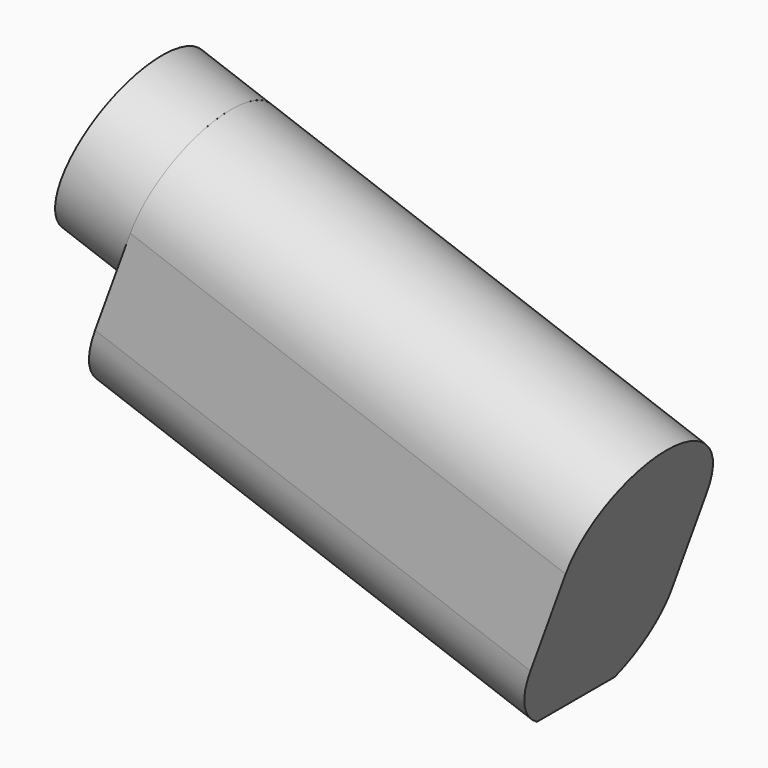
from build123d import *

# Parameters (mm, degrees)
F4_START = 63
F4_DEPTH = 10
F5_DEPTH = 63


# Not quite as in the source:
# - the program builds the solid bodies; features that only make, move or delete a surface that nothing else refers to are left out


with BuildPart() as f4:
    # F3 (on line) → F4 (new body)
    with BuildSketch(Plane(origin=(0, 0, 0), x_dir=(0, -1, 0), z_dir=(-0.9396926208, 0, 0.3420201433)).offset(F4_START)):
        with BuildLine():
            ThreePointArc((-12, 0), (0, -12), (12, 0))
            ThreePointArc((12, 0), (0, 12), (-12, 0))
        make_face()
    extrude(amount=F4_DEPTH)


with BuildPart() as f5:
    # F3 (on line) → F5 (new body)
    with BuildSketch(Plane(origin=(0, 0, 0), x_dir=(0, -1, 0), z_dir=(-0.9396926208, 0, 0.3420201433))):
        with BuildLine():
            Line((12, -14), (12, 0))
            ThreePointArc((12, 0), (0, -12), (-12, 0))
            Line((-12, 0), (-12, -14))
            ThreePointArc((-12, -14), (-10.5735281474, -19.6745486619), (-6.6332495807, -24))
            Line((-6.6332495807, -24), (6.6332495807, -24))
            ThreePointArc((6.6332495807, -24), (10.5735281474, -19.6745486619), (12, -14))
        make_face()
        with BuildLine():
            ThreePointArc((-12, 0), (0, -12), (12, 0))
            ThreePointArc((12, 0), (0, 12), (-12, 0))
        make_face()
    extrude(amount=F5_DEPTH)


solid = Compound([f4.part, f5.part])
